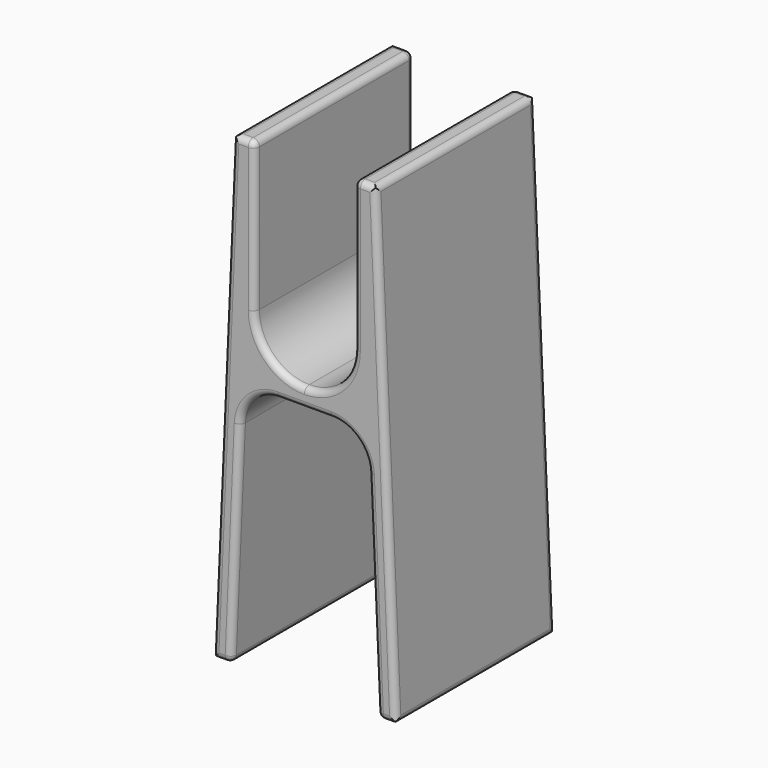
from build123d import *

# Parameters (mm, degrees)
F1_DEPTH     = 50.8
F2_R         = 1.5875
F3_T1_DEPTH  = 55.2235032041
F3_T3_DEPTH  = 55.9166206728
F4_T1_DEPTH  = 47.625
F4_T6_DEPTH  = 1.5875
F4_T12_DEPTH = 1.5875
F4_T18_DEPTH = 1.5875
F4_T24_DEPTH = 1.5875
F4_S29_W     = 1.5875
F4_S29_H     = 1.5875
F4_T30_DEPTH = 1.5875
F4_S35_W     = 1.5875
F4_S35_H     = 1.5875
F4_T36_DEPTH = 1.5875
F4_S41_W     = 1.5875
F4_S41_H     = 1.5875
F4_T42_DEPTH = 1.5875
F4_S47_W     = 1.5875
F4_S47_H     = 1.5875
F4_T48_DEPTH = 1.5875


# Not quite as in the source:
# - a fillet or chamfer that OpenCascade refuses, or shapes differently, is made with other operations: its cross-section is extruded or revolved along the edge and cut away or added


with BuildPart() as f1:
    # F0 (on Front) → F1 (new body)
    with BuildSketch(Plane.XZ):
        with BuildLine():
            Line((-18.2115888596, 55.5625), (-23.4099698747, -63.5))
            Line((-23.4099698747, -63.5), (-18.6474698747, -63.5))
            Line((-18.6474698747, -63.5), (-16.2727304656, -9.1095253353))
            ThreePointArc((-16.2727304656, -9.1095253353), (-13.3434580113, -2.6444832614), (-6.756796155, 0))
            Line((-6.756796155, 0), (0, 0))
            Line((0, 0), (0, 4.7625))
            ThreePointArc((0, 4.7625), (-8.9802561211, 8.4822438789), (-12.7, 17.4625))
            Line((-12.7, 17.4625), (-12.7, 55.5625))
            Line((-12.7, 55.5625), (-18.2115888596, 55.5625))
        make_face()
        with BuildLine():
            Line((0, 4.7625), (0, 0))
            Line((0, 0), (6.756796155, 0))
            ThreePointArc((6.756796155, 0), (13.3434580113, -2.6444832614), (16.2727304656, -9.1095253353))
            Line((16.2727304656, -9.1095253353), (18.6474698747, -63.5))
            Line((18.6474698747, -63.5), (23.4099698747, -63.5))
            Line((23.4099698747, -63.5), (18.2115888596, 55.5625))
            Line((18.2115888596, 55.5625), (12.7, 55.5625))
            Line((12.7, 55.5625), (12.7, 17.4625))
            ThreePointArc((12.7, 17.4625), (8.9802561211, 8.4822438789), (0, 4.7625))
        make_face()
    extrude(amount=F1_DEPTH)

    # F2
    f2_edges = [f1.edges().sort_by_distance(p)[0] for p in [
        (-20.810779, -50.8, -3.96875),
        (-21.02872, -50.8, -63.5),
        (-17.4601, -50.8, -36.304763),
        (-13.343458, -50.8, -2.644483),
        (0, -50.8, 0),
        (13.343458, -50.8, -2.644483),
        (17.4601, -50.8, -36.304763),
        (21.02872, -50.8, -63.5),
        (20.810779, -50.8, -3.96875),
        (15.455794, -50.8, 55.5625),
        (12.7, -50.8, 36.5125),
        (0, -50.8, 4.7625),
        (-12.7, -50.8, 36.5125),
        (-15.455794, -50.8, 55.5625),
        (-20.810779, 0, -3.96875),
        (-21.02872, 0, -63.5),
        (-17.4601, 0, -36.304763),
        (-13.343458, 0, -2.644483),
        (0, 0, 0),
        (13.343458, 0, -2.644483),
        (17.4601, 0, -36.304763),
        (21.02872, 0, -63.5),
        (20.810779, 0, -3.96875),
        (15.455794, 0, 55.5625),
        (12.7, 0, 36.5125),
        (0, 0, 4.7625),
        (-12.7, 0, 36.5125),
        (-15.455794, 0, 55.5625),
    ]]
    fillet(f2_edges, radius=F2_R)

    # F3: fillet of radius 1.5875 on 8 edges, made by hand

    # F3_s2 → F3_t1 (cut)
    with BuildSketch(Plane.XZ.offset(-2.2117516021)):
        with BuildLine():
            ThreePointArc((-18.2778772706, 54.0442457774), (-17.7896651949, 55.1217527898), (-16.6918882188, 55.5625))
            Line((-16.6918882188, 55.5625), (-18.2115888596, 55.5625))
            Line((-18.2115888596, 55.5625), (-18.2778772706, 54.0442457774))
        make_face()
        with BuildLine():
            ThreePointArc((16.6918882188, 55.5625), (17.7896651949, 55.1217527898), (18.2778772706, 54.0442457774))
            Line((18.2778772706, 54.0442457774), (18.2115888596, 55.5625))
            Line((18.2115888596, 55.5625), (16.6918882188, 55.5625))
        make_face()
    extrude(amount=F3_T1_DEPTH, mode=Mode.SUBTRACT)

    # F3_s4 → F3_t3 (cut)
    with BuildSketch(Plane.XZ.offset(-2.5583103364)):
        with BuildLine():
            ThreePointArc((-23.3376347919, -61.8432542226), (-22.8983985299, -63.0102769761), (-21.7516457401, -63.5))
            Line((-21.7516457401, -63.5), (-23.4099698747, -63.5))
            Line((-23.4099698747, -63.5), (-23.3376347919, -61.8432542226))
        make_face()
        with BuildLine():
            ThreePointArc((23.3376347919, -61.8432542226), (22.8983985299, -63.0102769761), (21.7516457401, -63.5))
            Line((21.7516457401, -63.5), (23.4099698747, -63.5))
            Line((23.4099698747, -63.5), (23.3376347919, -61.8432542226))
        make_face()
    extrude(amount=F3_T3_DEPTH, mode=Mode.SUBTRACT)

    # F4: fillet of radius 1.5875 on 4 edges, made by hand

    # F4_s2 → F4_t1 (cut)
    with BuildSketch(Plane.XZ.offset(1.5875)):
        with BuildLine():
            ThreePointArc((-14.2875, 55.5625), (-13.1649679849, 55.0975320151), (-12.7, 53.975))
            Line((-12.7, 53.975), (-12.7, 55.5625))
            Line((-12.7, 55.5625), (-14.2875, 55.5625))
        make_face()
        with BuildLine():
            ThreePointArc((12.7, 53.975), (13.1649679849, 55.0975320151), (14.2875, 55.5625))
            Line((14.2875, 55.5625), (12.7, 55.5625))
            Line((12.7, 55.5625), (12.7, 53.975))
        make_face()
        with BuildLine():
            ThreePointArc((-20.1671705155, -63.5), (-19.0693935395, -63.0592527898), (-18.5811814638, -61.9817457774))
            Line((-18.5811814638, -61.9817457774), (-18.6474698747, -63.5))
            Line((-18.6474698747, -63.5), (-20.1671705155, -63.5))
        make_face()
        with BuildLine():
            ThreePointArc((18.5811814638, -61.9817457774), (19.0693935395, -63.0592527898), (20.1671705155, -63.5))
            Line((20.1671705155, -63.5), (18.6474698747, -63.5))
            Line((18.6474698747, -63.5), (18.5811814638, -61.9817457774))
        make_face()
    extrude(amount=F4_T1_DEPTH, mode=Mode.SUBTRACT)


with BuildPart() as f4_tool4:
    # F4_s5 → F4_t6 (new body)
    with BuildSketch(Plane.XZ.offset(1.5875)):
        Polygon((20.1671705155, -61.9125), (18.5811814638, -61.9817457774), (18.6474698747, -63.5), (20.1671705155, -63.5), align=None)
    extrude(amount=-F4_T6_DEPTH)

    # F4_s7 → F4_t8 (revolve, cut)
    with BuildSketch(Plane(origin=(20.1671705155, -1.5875, -61.9125), x_dir=(0.6915130558, 0, 0.7223639621), z_dir=(-0.7223639621, 0, 0.6915130558))):
        with BuildLine():
            ThreePointArc((0, -1.5875), (1.5875, 0), (0, 1.5875))
            Line((0, 1.5875), (0, -1.5875))
        make_face()
    revolve(axis=Axis((20.1671705155, -1.5875, -61.9125), (0, 1, 0)), mode=Mode.SUBTRACT)


with BuildPart() as f1_1:
    add(f1.part)

    # F4_t3: cut F4_tool4
    add(f4_tool4.part, mode=Mode.SUBTRACT)


with BuildPart() as f4_tool10:
    # F4_s11 → F4_t12 (new body)
    with BuildSketch(Plane.XZ.offset(49.2125)):
        Polygon((20.1671705155, -61.9125), (18.5811814638, -61.9817457774), (18.6474698747, -63.5), (20.1671705155, -63.5), align=None)
    extrude(amount=F4_T12_DEPTH)

    # F4_s13 → F4_t14 (revolve, cut)
    with BuildSketch(Plane(origin=(20.1671705155, -49.2125, -61.9125), x_dir=(0.6915130558, 0, 0.7223639621), z_dir=(0.7223639621, 0, -0.6915130558))):
        with BuildLine():
            ThreePointArc((0, -1.5875), (1.5875, 0), (0, 1.5875))
            Line((0, 1.5875), (0, -1.5875))
        make_face()
    revolve(axis=Axis((20.1671705155, -49.2125, -61.9125), (0, -1, 0)), mode=Mode.SUBTRACT)


with BuildPart() as f1_2:
    add(f1_1.part)

    # F4_t9: cut F4_tool10
    add(f4_tool10.part, mode=Mode.SUBTRACT)


with BuildPart() as f4_tool16:
    # F4_s17 → F4_t18 (new body)
    with BuildSketch(Plane.XZ.offset(1.5875)):
        Polygon((-20.1671705155, -61.9125), (-20.1671705155, -63.5), (-18.6474698747, -63.5), (-18.5811814638, -61.9817457774), align=None)
    extrude(amount=-F4_T18_DEPTH)

    # F4_s19 → F4_t20 (revolve, cut)
    with BuildSketch(Plane(origin=(-20.1671705155, -1.5875, -61.9125), x_dir=(-0.6915130558, 0, 0.7223639621), z_dir=(-0.7223639621, 0, -0.6915130558))):
        with BuildLine():
            ThreePointArc((0, -1.5875), (1.5875, 0), (0, 1.5875))
            Line((0, 1.5875), (0, -1.5875))
        make_face()
    revolve(axis=Axis((-20.1671705155, -1.5875, -61.9125), (0, 1, 0)), mode=Mode.SUBTRACT)


with BuildPart() as f1_3:
    add(f1_2.part)

    # F4_t15: cut F4_tool16
    add(f4_tool16.part, mode=Mode.SUBTRACT)


with BuildPart() as f4_tool22:
    # F4_s23 → F4_t24 (new body)
    with BuildSketch(Plane.XZ.offset(49.2125)):
        Polygon((-20.1671705155, -61.9125), (-20.1671705155, -63.5), (-18.6474698747, -63.5), (-18.5811814638, -61.9817457774), align=None)
    extrude(amount=F4_T24_DEPTH)

    # F4_s25 → F4_t26 (revolve, cut)
    with BuildSketch(Plane(origin=(-20.1671705155, -49.2125, -61.9125), x_dir=(-0.6915130558, 0, 0.7223639621), z_dir=(0.7223639621, 0, 0.6915130558))):
        with BuildLine():
            ThreePointArc((0, -1.5875), (1.5875, 0), (0, 1.5875))
            Line((0, 1.5875), (0, -1.5875))
        make_face()
    revolve(axis=Axis((-20.1671705155, -49.2125, -61.9125), (0, -1, 0)), mode=Mode.SUBTRACT)


with BuildPart() as f1_4:
    add(f1_3.part)

    # F4_t21: cut F4_tool22
    add(f4_tool22.part, mode=Mode.SUBTRACT)


with BuildPart() as f4_tool28:
    # F4_s29 → F4_t30 (new body)
    with BuildSketch(Plane.YZ.offset(14.2875)):
        with Locations((-0.79375, 54.76875)):
            Rectangle(F4_S29_W, F4_S29_H)
    extrude(amount=-F4_T30_DEPTH)

    # F4_s31 → F4_t32 (revolve, cut)
    with BuildSketch(Plane(origin=(14.2875, -1.5875, 53.975), x_dir=(0, -0.7071067812, -0.7071067812), z_dir=(0, 0.7071067812, -0.7071067812))):
        with BuildLine():
            ThreePointArc((0, -1.5875), (1.5875, 0), (0, 1.5875))
            Line((0, 1.5875), (0, -1.5875))
        make_face()
    revolve(axis=Axis((14.2875, -1.5875, 53.975), (-1, 0, 0)), mode=Mode.SUBTRACT)


with BuildPart() as f1_5:
    add(f1_4.part)

    # F4_t27: cut F4_tool28
    add(f4_tool28.part, mode=Mode.SUBTRACT)


with BuildPart() as f4_tool34:
    # F4_s35 → F4_t36 (new body)
    with BuildSketch(Plane.YZ.offset(14.2875)):
        with Locations((-50.00625, 54.76875)):
            Rectangle(F4_S35_W, F4_S35_H)
    extrude(amount=-F4_T36_DEPTH)

    # F4_s37 → F4_t38 (revolve, cut)
    with BuildSketch(Plane(origin=(14.2875, -49.2125, 53.975), x_dir=(0, 0.7071067812, -0.7071067812), z_dir=(0, 0.7071067812, 0.7071067812))):
        with BuildLine():
            ThreePointArc((0, -1.5875), (1.5875, 0), (0, 1.5875))
            Line((0, 1.5875), (0, -1.5875))
        make_face()
    revolve(axis=Axis((14.2875, -49.2125, 53.975), (-1, 0, 0)), mode=Mode.SUBTRACT)


with BuildPart() as f1_6:
    add(f1_5.part)

    # F4_t33: cut F4_tool34
    add(f4_tool34.part, mode=Mode.SUBTRACT)


with BuildPart() as f4_tool40:
    # F4_s41 → F4_t42 (new body)
    with BuildSketch(Plane.XY.offset(53.975)):
        with Locations((-13.49375, -0.79375)):
            Rectangle(F4_S41_W, F4_S41_H)
    extrude(amount=F4_T42_DEPTH)

    # F4_s43 → F4_t44 (revolve, cut)
    with BuildSketch(Plane(origin=(-14.2875, -1.5875, 53.975), x_dir=(-0.7071067812, -0.7071067812, 0), z_dir=(-0.7071067812, 0.7071067812, 0))):
        with BuildLine():
            ThreePointArc((0, -1.5875), (1.5875, 0), (0, 1.5875))
            Line((0, 1.5875), (0, -1.5875))
        make_face()
    revolve(axis=Axis((-14.2875, -1.5875, 53.975), (0, 0, 1)), mode=Mode.SUBTRACT)


with BuildPart() as f1_7:
    add(f1_6.part)

    # F4_t39: cut F4_tool40
    add(f4_tool40.part, mode=Mode.SUBTRACT)


with BuildPart() as f4_tool46:
    # F4_s47 → F4_t48 (new body)
    with BuildSketch(Plane.XY.offset(53.975)):
        with Locations((-13.49375, -50.00625)):
            Rectangle(F4_S47_W, F4_S47_H)
    extrude(amount=F4_T48_DEPTH)

    # F4_s49 → F4_t50 (revolve, cut)
    with BuildSketch(Plane(origin=(-14.2875, -49.2125, 53.975), x_dir=(-0.7071067812, 0.7071067812, 0), z_dir=(0.7071067812, 0.7071067812, 0))):
        with BuildLine():
            ThreePointArc((0, -1.5875), (1.5875, 0), (0, 1.5875))
            Line((0, 1.5875), (0, -1.5875))
        make_face()
    revolve(axis=Axis((-14.2875, -49.2125, 53.975), (0, 0, 1)), mode=Mode.SUBTRACT)


with BuildPart() as f1_8:
    add(f1_7.part)

    # F4_t45: cut F4_tool46
    add(f4_tool46.part, mode=Mode.SUBTRACT)


solid = f1_8.part
